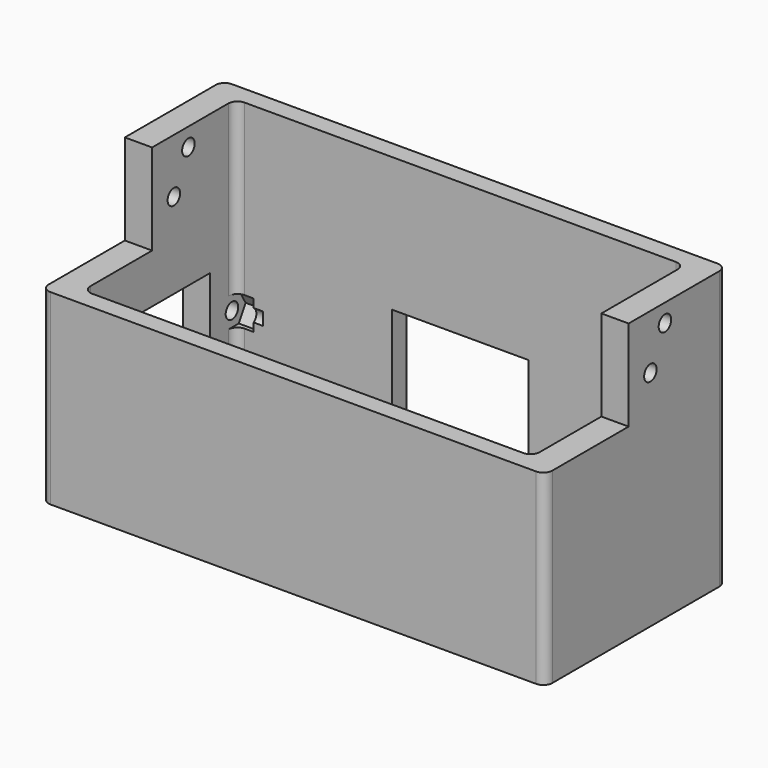
from build123d import *

# Parameters (mm, degrees)
F0_W      = 111
F0_H      = 50
F0_W_2    = 99
F0_H_2    = 42
F1_DEPTH  = 1.2
F2_DEPTH  = 41.2
F3_W      = 30.1
F3_H      = 22
F4_DEPTH  = 4
F6_DEPTH  = 20
F7_R      = 1.725
F8_DEPTH  = 114.6
F7_W      = 28
F7_H      = 19.5
F9_DEPTH  = 12
F11_DEPTH = 4
F12_R     = 2


# Not quite as in the source:
# - a feature names something its author has since deleted; it is built from what else it names


with BuildPart() as f1:
    # F0 (on Top) → F1 (new body)
    with BuildSketch(Plane.XY):
        with Locations((55.5, 25)):
            Rectangle(F0_W, F0_H)
        with Locations((55.5, 25)):
            Rectangle(F0_W_2, F0_H_2, mode=Mode.SUBTRACT)
        with Locations((55.5, 25)):
            Rectangle(F0_W_2, F0_H_2)
        with BuildLine():
            ThreePointArc((25.5, 13), (26.9644660941, 16.5355339059), (30.5, 18))
            Line((30.5, 18), (80.5, 18))
            ThreePointArc((80.5, 18), (84.0355339059, 16.5355339059), (85.5, 13))
            Line((85.5, 13), (85.5, 11))
            ThreePointArc((85.5, 11), (84.0355339059, 7.4644660941), (80.5, 6))
            Line((80.5, 6), (30.5, 6))
            ThreePointArc((30.5, 6), (26.9644660941, 7.4644660941), (25.5, 11))
            Line((25.5, 11), (25.5, 13))
        make_face(mode=Mode.SUBTRACT)
    extrude(amount=F1_DEPTH)

    # F0 (on Top) → F2 (join)
    with BuildSketch(Plane.XY):
        with Locations((55.5, 25)):
            Rectangle(F0_W, F0_H)
        with Locations((55.5, 25)):
            Rectangle(F0_W_2, F0_H_2, mode=Mode.SUBTRACT)
    extrude(amount=F2_DEPTH)

    # F3 (on face) → F4 (cut)
    with BuildSketch(Plane(origin=(0, 50, 0), x_dir=(-1, 0, 0), z_dir=(0, 1, 0))):
        with Locations((-55.5, 20.6)):
            Rectangle(F3_W, F3_H)
    extrude(amount=-F4_DEPTH, mode=Mode.SUBTRACT)

    # F5 (on face) → F6 (join)
    with BuildSketch(Plane.XY.offset(41.2)):
        Polygon((0, 50), (0, 23), (6, 23), (6, 46), (105, 46), (105, 23), (111, 23), (111, 50), align=None)
    extrude(amount=F6_DEPTH)

    # F7 (on face) → F8 (cut)
    with BuildSketch(Plane(origin=(0, 0, 0), x_dir=(0, -1, 0), z_dir=(-1, 0, 0))):
        with Locations((-29, 49.2)):
            Circle(F7_R)
        with Locations((-33, 57.2)):
            Circle(F7_R)
    extrude(amount=-F8_DEPTH, mode=Mode.SUBTRACT)

    # F7 (on face) → F9 (cut)
    with BuildSketch(Plane(origin=(0, 0, 0), x_dir=(0, -1, 0), z_dir=(-1, 0, 0))):
        with Locations((-25, 20.6)):
            Rectangle(F7_W, F7_H)
        with Locations((-45, 20.6)):
            Circle(F7_R)
        with Locations((-5, 20.6)):
            Circle(F7_R)
    extrude(amount=-F9_DEPTH, mode=Mode.SUBTRACT)

    # F10 (on face) → F11 (cut)
    with BuildSketch(Plane.YZ.offset(6)):
        Polygon((8.7527767497, 20.6), (6.8763883749, 23.85), (3.1236116251, 23.85), (1.2472232503, 20.6), (3.1236116251, 17.35), (6.8763883749, 17.35), align=None)
        Polygon((43.1236116251, 23.85), (41.2472232503, 20.6), (43.1236116251, 17.35), (46.8763883749, 17.35), (48.7527767497, 20.6), (46.8763883749, 23.85), align=None)
    extrude(amount=F11_DEPTH, mode=Mode.SUBTRACT)

    # F12
    f12_edges = [f1.edges().sort_by_distance(p)[0] for p in [
        (6, 46, 42.525),
        (6, 46, 9.275),
        (105, 46, 31.2),
        (105, 4, 21.2),
        (6, 4, 32.525),
        (6, 4, 9.275),
        (111, 0, 20.6),
        (111, 50, 30.6),
        (0, 50, 30.6),
        (0, 0, 20.6),
    ]]
    fillet(f12_edges, radius=F12_R)


solid = f1.part
